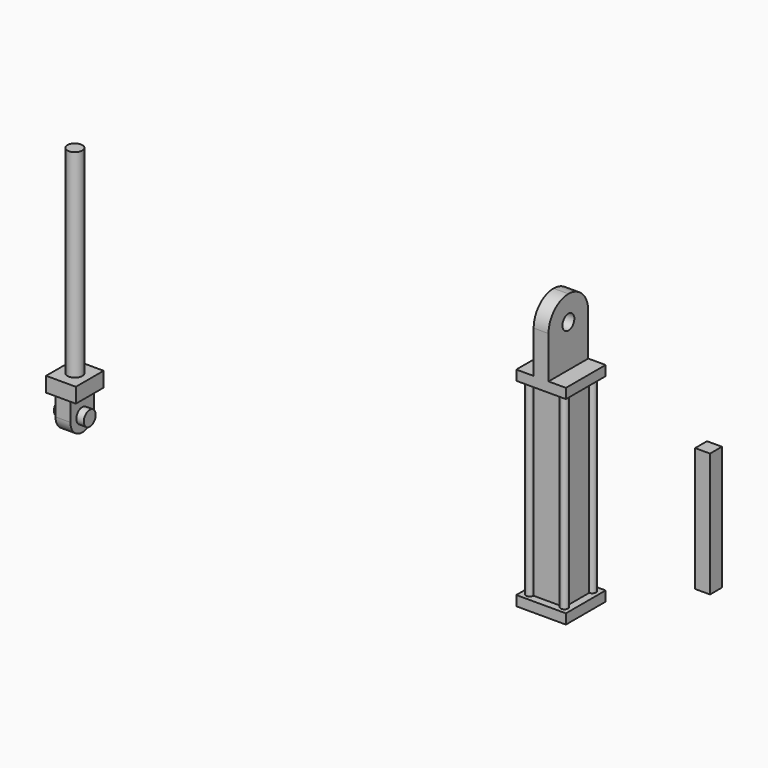
from build123d import *

# Parameters (mm, degrees)
F0_W           = 2.54
F0_H           = 2.54
F1_DEPTH       = 0.508
F3_R           = 0.1905
F2_W           = 1.778
F2_H           = 1.778
F4_DEPTH       = 9.652
F5_W           = 2.54
F5_H           = 2.54
F6_DEPTH       = 0.508
F7_W           = 0.762
F7_H           = 2.54
F8_DEPTH       = 3.429
F9_R           = 1.26999
F10_R          = 0.381
F11_DEPTH      = 10.16
F12_W          = 1.524
F12_H          = 1.778
F13_DEPTH      = 0.762
F14_R          = 0.381
F15_DEPTH      = 10.16
F16_W          = 0.762
F16_H          = 1.524
F17_DEPTH      = 1.778
F18_R          = 0.76199
F20_R          = 0.381
F21_DEPTH      = 0.381
F21_DEPTH_BACK = 1.143
F19_R          = 0.381
F22_DEPTH      = 0.762
F23_W          = 0.762
F23_H          = 5.08
F24_DEPTH      = 0.762


# Not quite as in the source:
# - a fillet or chamfer is up to 0.001 mm smaller than in the source, because OpenCascade refuses the exact size
# - a pattern or mirror of a feature is missing from the dataset's text; its kind, count and spacing are read off the source's solid
# - a feature names something its author has since deleted; it is built from what else it names


with BuildPart() as f1:
    # F0 (on Top) → F1 (new body)
    with BuildSketch(Plane.XY):
        with Locations((-1.27, 1.27)):
            Rectangle(F0_W, F0_H)
    extrude(amount=F1_DEPTH)

    # F3 (on face) + F2 (on face) → F4 (join)
    with BuildSketch(Plane.XY.offset(0.508)):
        with Locations((-2.159, 0.381)):
            Circle(F3_R)
        with Locations((-0.381, 0.381)):
            Circle(F3_R)
        with Locations((-0.381, 2.159)):
            Circle(F3_R)
        with Locations((-2.159, 2.159)):
            Circle(F3_R)
    with BuildSketch(Plane.XY.offset(0.508)):
        with Locations((-1.27, 1.27)):
            Rectangle(F2_W, F2_H)
    extrude(amount=F4_DEPTH)

    # F5 (on face) → F6 (join)
    with BuildSketch(Plane.XY.offset(10.16)):
        with Locations((-1.27, 1.27)):
            Rectangle(F5_W, F5_H)
    extrude(amount=F6_DEPTH)

    # F7 (on face) → F8 (join)
    with BuildSketch(Plane.XY.offset(10.668)):
        with Locations((-1.27, 1.27)):
            Rectangle(F7_W, F7_H)
    extrude(amount=F8_DEPTH)

    # F9 (radius 1.27 in the source; OpenCascade refuses exactly that, so slightly less here)
    f9_edges = [f1.edges().sort_by_distance(p)[0] for p in [
        (-1.27, 0, 14.097),
        (-1.27, 2.54, 14.097),
    ]]
    fillet(f9_edges, radius=F9_R)

    # F10 (on face) → F11 (cut)
    with BuildSketch(Plane(origin=(0, 0, 0), x_dir=(1, 0, 0), z_dir=(0, 0, -1))):
        with Locations((-1.27, -1.27)):
            Circle(F10_R)
    extrude(amount=-F11_DEPTH, mode=Mode.SUBTRACT)

    # F19 (on face) → F22 (cut)
    with BuildSketch(Plane.YZ.offset(-0.889)):
        with Locations((1.27, 12.827)):
            Circle(F19_R)
    extrude(amount=-F22_DEPTH, mode=Mode.SUBTRACT)


with BuildPart() as f13:
    # F12 (on Top) → F13 (new body)
    with BuildSketch(Plane.XY):
        with Locations((-28.0019982215, 3.5851696832)):
            Rectangle(F12_W, F12_H)
    extrude(amount=F13_DEPTH)

    # F14 (on face) → F15 (join)
    with BuildSketch(Plane.XY.offset(0.762)):
        with Locations((-28.0019982215, 3.5851696832)):
            Circle(F14_R)
    extrude(amount=F15_DEPTH)

    # F16 (on face) → F17 (join)
    with BuildSketch(Plane(origin=(0, 0, 0), x_dir=(1, 0, 0), z_dir=(0, 0, -1))):
        with Locations((-28.0019982215, -3.5851696832)):
            Rectangle(F16_W, F16_H)
    extrude(amount=F17_DEPTH)

    # F18 (radius 0.762 in the source; OpenCascade refuses exactly that, so slightly less here)
    f18_edges = [f13.edges().sort_by_distance(p)[0] for p in [
        (-28.001998, 2.82317, -1.778),
        (-28.001998, 4.34717, -1.778),
    ]]
    fillet(f18_edges, radius=F18_R)

    # F20 (on face) → F21 (join, two sides)
    with BuildSketch(Plane.YZ.offset(-27.6209982215)) as f21_sk:
        with Locations((3.5851696832, -1.016)):
            Circle(F20_R)
    extrude(amount=F21_DEPTH)
    extrude(f21_sk.sketch, amount=-F21_DEPTH_BACK)


with BuildPart() as f24:
    # F23 (on Front) → F24 (new body)
    with BuildSketch(Plane.XZ):
        with Locations((7.6038887042, 6.803626753)):
            Rectangle(F23_W, F23_H)
    extrude(amount=F24_DEPTH)

    # F24_copies: F24 across plane


with BuildPart() as f24_1:
    add(f24.part)
    add(f24.part.mirror(Plane.XY.offset(7.438627)))


solid = Compound([f1.part, f13.part, f24_1.part])
